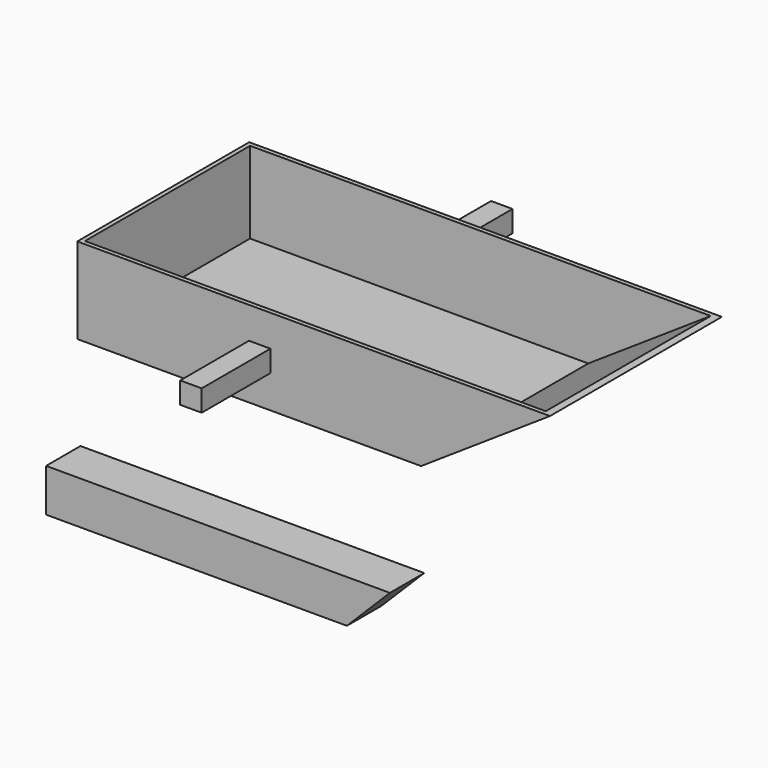
from build123d import *

# Parameters (mm, degrees)
F0_W     = 203.2
F0_H     = 50.8
F1_DEPTH = 3.175
F4_DEPTH = 63.5
F5_T     = -2.54
F6_W     = 50.8
F6_H     = 12.7
F7_DEPTH = 12.7
F8_W     = 177.8
F8_H     = 25.4
F9_DEPTH = 25.4


with BuildPart() as f1:
    # F0 (on Front) → F1 (new body, symmetric)
    with BuildSketch(Plane.XZ):
        Polygon((177.8, 25.4), (101.6, 25.4), (101.6, -25.4), align=None)
        Rectangle(F0_W, F0_H)
    extrude(amount=F1_DEPTH, both=True)


with BuildPart() as f2_1:
    # F2: copy of F1
    add(f1.part)


with BuildPart() as f1_1:
    add(f1.part)

    # F4 (add, symmetric): a face of the model
    f4_faces = [f1_1.faces().sort_by_distance(p)[0] for p in [
        (20.0526315789, -3.175, 1.3368421053),
    ]]
    extrude(f4_faces, amount=F4_DEPTH, both=True)

    # F5
    f5_openings = [f1_1.faces().sort_by_distance(p)[0] for p in [
        (38.1, -3.175, 25.4),
    ]]
    offset(amount=F5_T, openings=f5_openings)


with BuildPart() as f7:
    # F6 (on Right) → F7 (new body)
    with BuildSketch(Plane.YZ):
        with Locations((-92.2398825281, 0.4846053965)):
            Rectangle(F6_W, F6_H)
    extrude(amount=F7_DEPTH)


with BuildPart() as f7b:
    # F6 (on Right) → F7, piece 2 (new body)
    with BuildSketch(Plane.YZ):
        with Locations((86.6106621265, 0.4846053965)):
            Rectangle(F6_W, F6_H)
    extrude(amount=F7_DEPTH)


with BuildPart() as f9:
    # F8 (on Front) → F9 (new body)
    with BuildSketch(Plane.XZ):
        Polygon((50.1418564967, -124.886709961), (24.7418564967, -124.886709961), (24.7418564967, -150.286709961), align=None)
        with Locations((-64.1581435033, -137.586709961)):
            Rectangle(F8_W, F8_H)
    extrude(amount=F9_DEPTH)


solid = Compound([f1_1.part, f7.part, f7b.part, f9.part])
